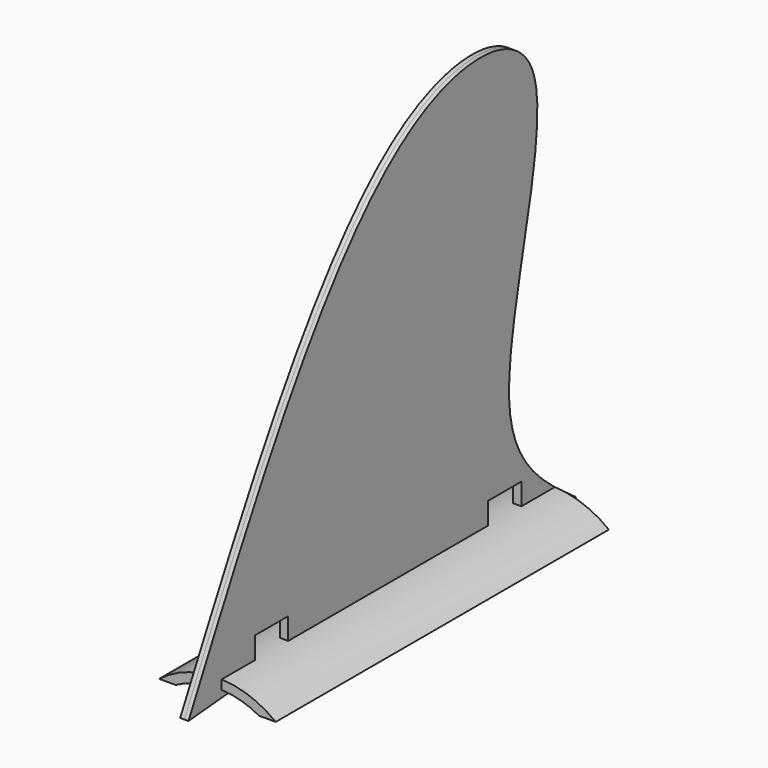
from build123d import *

# Parameters (mm, degrees)
F2_DEPTH = 25
F3_DEPTH = 0.5
F4_W     = 5
F4_H     = 3
F5_DEPTH = 1


with BuildPart() as f2:
    # F0 (on Front) → F2 (new body, symmetric)
    with BuildSketch(Plane.XZ):
        with BuildLine():
            ThreePointArc((-5, 0), (0, 1.295630141), (5, 0))
            Line((5, 0), (7, 0))
            ThreePointArc((7, 0), (0, 2.401754251), (-7, 0))
            Line((-7, 0), (-5, 0))
        make_face()
    extrude(amount=F2_DEPTH, both=True)


with BuildPart() as f3:
    # F1 (on Right) → F3 (new body, symmetric)
    with BuildSketch(Plane.YZ):
        with BuildLine():
            add(Edge.make_bspline(
                [(-29.968450375, 0), (-20.2834898441, 0.8980619755), (-0.9008219888, 2.6953679045), (18.52041614, 0.8988497881), (28.2374212838, 0)],
                knots=[0, 0, 0, 0, 0.4996711806, 1, 1, 1, 1], degree=3))
            add(Edge.make_bspline(
                [(28.2374212838, 0), (23.5346273127, 3.3426593215), (12.1004134849, 11.4698878734), (29.9820999442, 52.4786254251), (-2.1355902035, 54.384946251), (-18.9209685078, 21.5865959824), (-29.968450375, 0)],
                knots=[0, 0, 0, 0, 0.1878770554, 0.456797903, 0.6424855486, 1, 1, 1, 1], degree=3))
        make_face()
    extrude(amount=F3_DEPTH, both=True)

    # F4 (on Right) → F5 (cut, symmetric)
    with BuildSketch(Plane.YZ):
        with Locations((-17.5, 3.5)):
            Rectangle(F4_W, F4_H)
        with Locations((17.5, 3.5)):
            Rectangle(F4_W, F4_H)
    extrude(amount=F5_DEPTH, both=True, mode=Mode.SUBTRACT)


solid = Compound([f2.part, f3.part])
